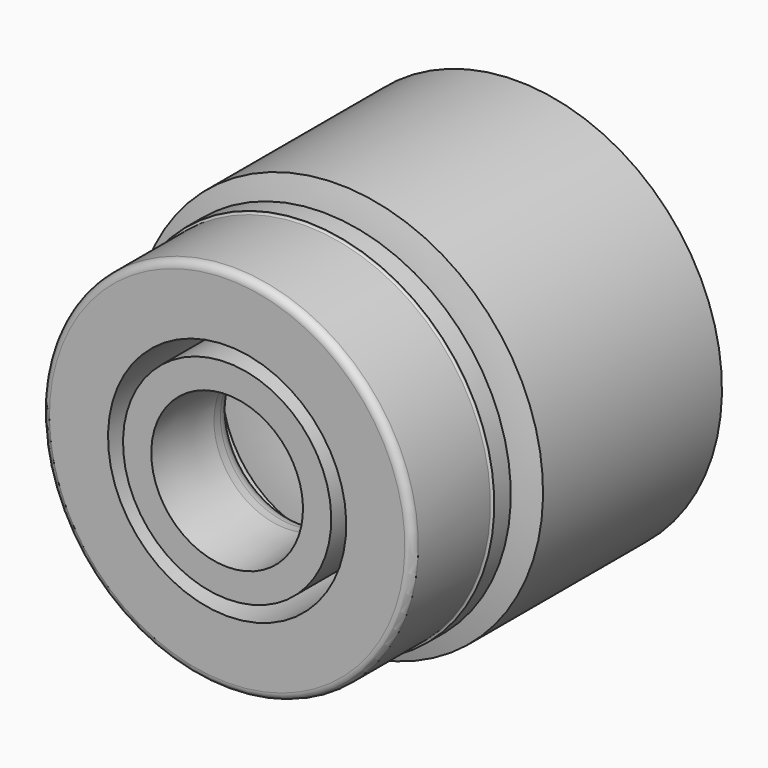
from build123d import *


# Not quite as in the source:
# - ends of sketch curves that miss each other by under 0.0002 mm in the source are joined


with BuildPart() as f1:
    # F0 (on Right) → F1 (revolve)
    with BuildSketch(Plane.YZ):
        with BuildLine():
            Line((48.3, 0), (44.8, 0))
            Line((44.8, 0), (44.8, -13.875))
            Line((44.8, -13.875), (44.8, -15.875))
            Line((44.8, -15.875), (44.8, -16))
            Line((44.8, -16), (50.2419314905, -16))
            ThreePointArc((50.2419314905, -16), (49.9533733583, -7.9171756979), (48.3, 0))
        make_face()
        with BuildLine():
            Line((44.8, -15.875), (16.5520520108, -15.875))
            ThreePointArc((16.5520520108, -15.875), (17.1768581598, -21.6470326742), (18.5, -27.3))
            Line((18.5, -27.3), (48.3, -27.3))
            ThreePointArc((48.3, -27.3), (49.6125845395, -21.7087079906), (50.2419314905, -16))
            Line((50.2419314905, -16), (44.8, -16))
            Line((44.8, -16), (44.8, -15.875))
        make_face()
        with BuildLine():
            Line((44.8, 0), (18.5, 0))
            ThreePointArc((18.5, 0), (16.9864772631, -6.8634600623), (16.5005319947, -13.875))
            Line((16.5005319947, -13.875), (44.8, -13.875))
            Line((44.8, -13.875), (44.8, 0))
        make_face()
    revolve(axis=Axis((0, 182.171996, 0), (0, 1, 0)))


with BuildPart() as f1b:
    # F0 (on Right) → F1, piece 2 (revolve)
    with BuildSketch(Plane.YZ):
        with BuildLine():
            Line((0, -13.875), (12.9311627863, -13.875))
            ThreePointArc((12.9311627863, -13.875), (13.1689777764, -13.2846144071), (13.25, -12.653309))
            Line((13.25, -12.653309), (13.25, -12.141094))
            ThreePointArc((13.25, -12.141094), (12.5790376496, -10.4367990501), (10.926302979, -9.6473182965))
            Line((10.926302979, -9.6473182965), (9.7628490509, -9.5650652795))
            Line((9.7628490509, -9.5650652795), (0, -10.10706))
            Line((0, -10.10706), (0, -13.875))
        make_face()
    revolve(axis=Axis((0, 182.171996, 0), (0, 1, 0)))


with BuildPart() as f1c:
    # F0 (on Right) → F1, piece 3 (revolve)
    with BuildSketch(Plane.YZ):
        with BuildLine():
            Line((16, -25), (16, -15.875))
            Line((16, -15.875), (0, -15.875))
            Line((0, -15.875), (0, -23.677925))
            ThreePointArc((0, -23.677925), (0.2928932188, -24.3850317812), (1, -24.677925))
            Line((1, -24.677925), (13, -24.677925))
            ThreePointArc((13, -24.677925), (13.1767766953, -24.7511483047), (13.25, -24.927925))
            Line((13.25, -24.927925), (13.25, -25))
            Line((13.25, -25), (16, -25))
        make_face()
    revolve(axis=Axis((0, 182.171996, 0), (0, 1, 0)))


solid = Compound([f1.part, f1b.part, f1c.part])
